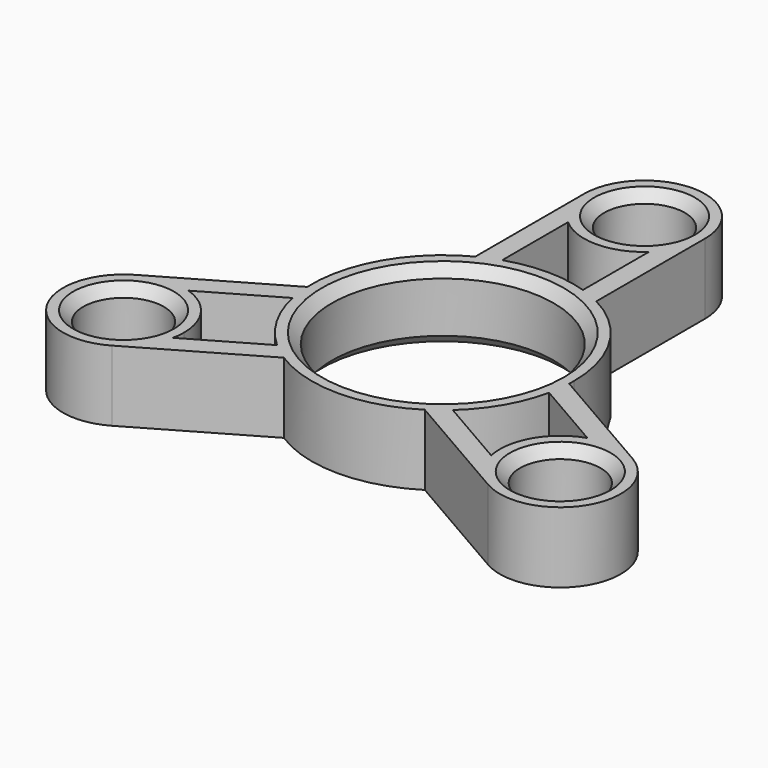
from build123d import *

# Parameters (mm, degrees)
F0_R     = 11
F0_R_2   = 4
F1_DEPTH = 3.5
F2_SIZE  = 1
F4_DEPTH = 7.001


# Not quite as in the source:
# - a feature names something its author has since deleted; it is built from what else it names


with BuildPart() as f1:
    # F0 (on Top) → F1 (new body, symmetric)
    with BuildSketch(Plane.XY):
        with BuildLine():
            ThreePointArc((-6, 11.5325625947), (0, 13), (6, 11.5325625947))
            Line((6, 11.5325625947), (6, 25))
            ThreePointArc((6, 25), (0, 19), (-6, 25))
            Line((-6, 25), (-6, 11.5325625947))
        make_face()
        with BuildLine():
            ThreePointArc((-6.9874921777, -10.96243372), (-11.2583302492, -6.5), (-12.9874921777, -0.5701288746))
            Line((-12.9874921777, -0.5701288746), (-24.6506350946, -7.3038475773))
            ThreePointArc((-24.6506350946, -7.3038475773), (-18.6506350946, -7.3038475773), (-15.6506350946, -12.5))
            ThreePointArc((-15.6506350946, -12.5), (-16.4544826719, -15.5), (-18.6506350946, -17.6961524227))
            Line((-18.6506350946, -17.6961524227), (-6.9874921777, -10.96243372))
        make_face()
        with BuildLine():
            Line((24.6506350946, -7.3038475773), (12.9874921777, -0.5701288746))
            ThreePointArc((12.9874921777, -0.5701288746), (11.2583302492, -6.5), (6.9874921777, -10.96243372))
            Line((6.9874921777, -10.96243372), (18.6506350946, -17.6961524227))
            ThreePointArc((18.6506350946, -17.6961524227), (16.4544826719, -9.5), (24.6506350946, -7.3038475773))
        make_face()
        with BuildLine():
            ThreePointArc((12.9874921777, -0.5701288746), (12.9968726683, -0.2851330301), (13, 0))
            ThreePointArc((13, 0), (11.1130553854, 6.7453687816), (6, 11.5325625947))
            ThreePointArc((6, 11.5325625947), (0, 13), (-6, 11.5325625947))
            ThreePointArc((-6, 11.5325625947), (-11.2583302492, 6.5), (-12.9874921777, -0.5701288746))
            ThreePointArc((-12.9874921777, -0.5701288746), (-11.2583302492, -6.5), (-6.9874921777, -10.96243372))
            ThreePointArc((-6.9874921777, -10.96243372), (0, -13), (6.9874921777, -10.96243372))
            ThreePointArc((6.9874921777, -10.96243372), (11.2583302492, -6.5), (12.9874921777, -0.5701288746))
        make_face()
        Circle(F0_R, mode=Mode.SUBTRACT)
        with BuildLine():
            ThreePointArc((-6, 25), (0, 19), (6, 25))
            ThreePointArc((6, 25), (0, 31), (-6, 25))
        make_face()
        with Locations((0, 25)):
            Circle(F0_R_2, mode=Mode.SUBTRACT)
        with BuildLine():
            ThreePointArc((-15.6506350946, -12.5), (-18.6506350946, -7.3038475773), (-24.6506350946, -7.3038475773))
            ThreePointArc((-24.6506350946, -7.3038475773), (-26.8467875173, -15.5), (-18.6506350946, -17.6961524227))
            ThreePointArc((-18.6506350946, -17.6961524227), (-16.4544826719, -15.5), (-15.6506350946, -12.5))
        make_face()
        with Locations((-21.6506350946, -12.5)):
            Circle(F0_R_2, mode=Mode.SUBTRACT)
        with BuildLine():
            ThreePointArc((27.6506350946, -12.5), (26.8467875173, -9.5), (24.6506350946, -7.3038475773))
            ThreePointArc((24.6506350946, -7.3038475773), (16.4544826719, -9.5), (18.6506350946, -17.6961524227))
            ThreePointArc((18.6506350946, -17.6961524227), (24.6506350946, -17.6961524227), (27.6506350946, -12.5))
        make_face()
        with Locations((21.6506350946, -12.5)):
            Circle(F0_R_2, mode=Mode.SUBTRACT)
    extrude(amount=F1_DEPTH, both=True)

    # F2
    f2_edges = [f1.edges().sort_by_distance(p)[0] for p in [
        (-4, 25, 3.5),
        (-11, 0, 3.5),
        (-25.650635, -12.5, 3.5),
        (17.650635, -12.5, 3.5),
        (-25.650635, -12.5, -3.5),
        (-11, 0, -3.5),
        (17.650635, -12.5, -3.5),
        (-4, 25, -3.5),
    ]]
    chamfer(f2_edges, length=F2_SIZE)

    # F3 (on face) → F4 (cut, through all)
    with BuildSketch(Plane.XY.offset(3.5)):
        with BuildLine():
            Line((4, 12.3693168769), (4, 20.527864045))
            ThreePointArc((4, 20.527864045), (0, 19), (-4, 20.527864045))
            Line((-4, 20.527864045), (-4, 12.3693168769))
            ThreePointArc((-4, 12.3693168769), (0, 13), (4, 12.3693168769))
        make_face()
        with BuildLine():
            ThreePointArc((-8.7121426428, -9.6487600536), (-11.2583302492, -6.5), (-12.7121426428, -2.7205568233))
            Line((-12.7121426428, -2.7205568233), (-19.7776517484, -6.7998304074))
            ThreePointArc((-19.7776517484, -6.7998304074), (-16.7907019635, -8.9813283811), (-15.6506350946, -12.5))
            ThreePointArc((-15.6506350946, -12.5), (-15.682473733, -13.117292444), (-15.7776517484, -13.7280336376))
            Line((-15.7776517484, -13.7280336376), (-8.7121426428, -9.6487600536))
        make_face()
        with BuildLine():
            Line((19.7776517484, -6.7998304074), (12.7121426428, -2.7205568233))
            ThreePointArc((12.7121426428, -2.7205568233), (11.2583302492, -6.5), (8.7121426428, -9.6487600536))
            Line((8.7121426428, -9.6487600536), (15.7776517484, -13.7280336376))
            ThreePointArc((15.7776517484, -13.7280336376), (16.4544826719, -9.5), (19.7776517484, -6.7998304074))
        make_face()
    extrude(amount=-F4_DEPTH, mode=Mode.SUBTRACT)


solid = f1.part
